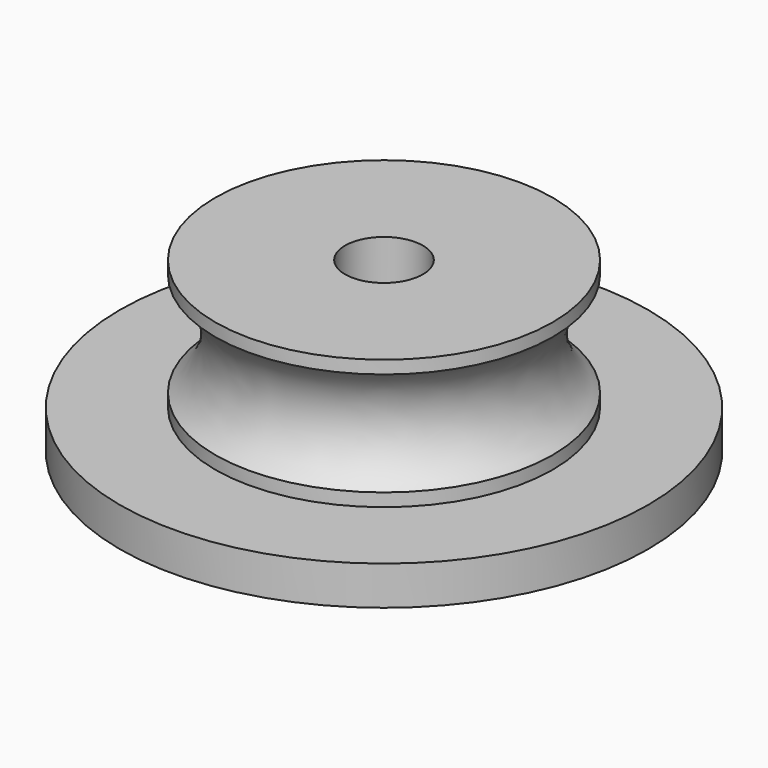
from build123d import *
from build123d import SkipClean  # not in build123d's __all__

# Parameters (mm, degrees)
F2_R     = 20.3469556015
F2_R_2   = 13
F2_R_3   = 3
F3_DEPTH = 3


with BuildPart() as f1:
    # F0 (on Right) → F1 (revolve)
    with BuildSketch(Plane.YZ):
        with BuildLine():
            Line((-3, -5), (-3, 0))
            Line((-3, 0), (-3, 5))
            Line((-3, 5), (-13, 5))
            Line((-13, 5), (-13, 4))
            ThreePointArc((-13, 4), (-11, 0), (-13, -4))
            Line((-13, -4), (-13, -5))
            Line((-13, -5), (-3, -5))
        make_face()
    revolve(axis=Axis((0, 0, 3.2237173374), (0, 0, 1)))

    # F2 (on face) → F3 (join)
    with BuildSketch(Plane(origin=(0, 0, -5), x_dir=(1, 0, 0), z_dir=(0, 0, -1))):
        Circle(F2_R)
        Circle(F2_R_2, mode=Mode.SUBTRACT)
        Circle(F2_R_2)
        Circle(F2_R_3, mode=Mode.SUBTRACT)
    with SkipClean():  # cleaning this boolean's faces spoils the solid; the shape is the same uncleaned
        extrude(amount=F3_DEPTH)


solid = f1.part
